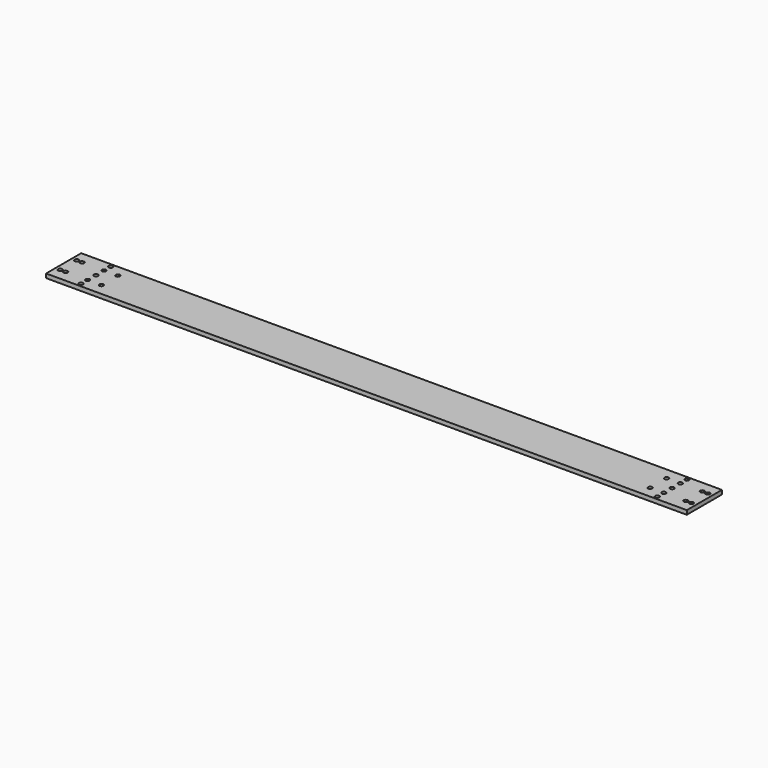
from build123d import *

# Parameters (mm, degrees)
F0_W     = 467
F0_H     = 32
F0_W_2   = 400
F0_H_2   = 15
F0_W_3   = 16
F0_W_4   = 10
F0_W_5   = 4
F1_DEPTH = 3
F2_D     = 3


# Not quite as in the source:
# - a feature names something its author has since deleted; it is built from what else it names


with BuildPart() as f1:
    # F0 (on Top) → F1 (new body)
    with BuildSketch(Plane.XY):
        Rectangle(F0_W, F0_H)
        Polygon((226, -7.5), (210, -7.5), (200, -7.5), (-200, -7.5), (-210, -7.5), (-226, -7.5), (-230, -7.5), (-230, 7.5), (-226, 7.5), (-210, 7.5), (-200, 7.5), (200, 7.5), (210, 7.5), (226, 7.5), (230, 7.5), (230, -7.5), align=None, mode=Mode.SUBTRACT)
        Rectangle(F0_W_2, F0_H_2)
        with Locations((218, 0)):
            Rectangle(F0_W_3, F0_H_2)
        with Locations((-218, 0)):
            Rectangle(F0_W_3, F0_H_2)
        with Locations((205, 0)):
            Rectangle(F0_W_4, F0_H_2)
        with Locations((-205, 0)):
            Rectangle(F0_W_4, F0_H_2)
        with Locations((-228, 0)):
            Rectangle(F0_W_5, F0_H_2)
        with Locations((228, 0)):
            Rectangle(F0_W_5, F0_H_2)
    extrude(amount=F1_DEPTH)

    # F2 (through all)
    with Locations(Plane(origin=(0, 0, 0), x_dir=(1, 0, 0), z_dir=(0, 0, -1))):
        with Locations((210, 7.5), (210, -7.5), (230, -7.5), (230, 7.5), (-210, 7.5), (-210, -7.5), (-230, -7.5), (-230, 7.5), (210, 13.5), (-210, 13.5), (-210, -13.5), (210, -13.5), (226, 7.5), (226, -7.5), (-226, 7.5), (-226, -7.5), (200, 7.5), (200, -7.5), (-200, -7.5), (-200, 7.5), (-210, 0), (210, 0)):
            Hole(F2_D / 2)


solid = f1.part
